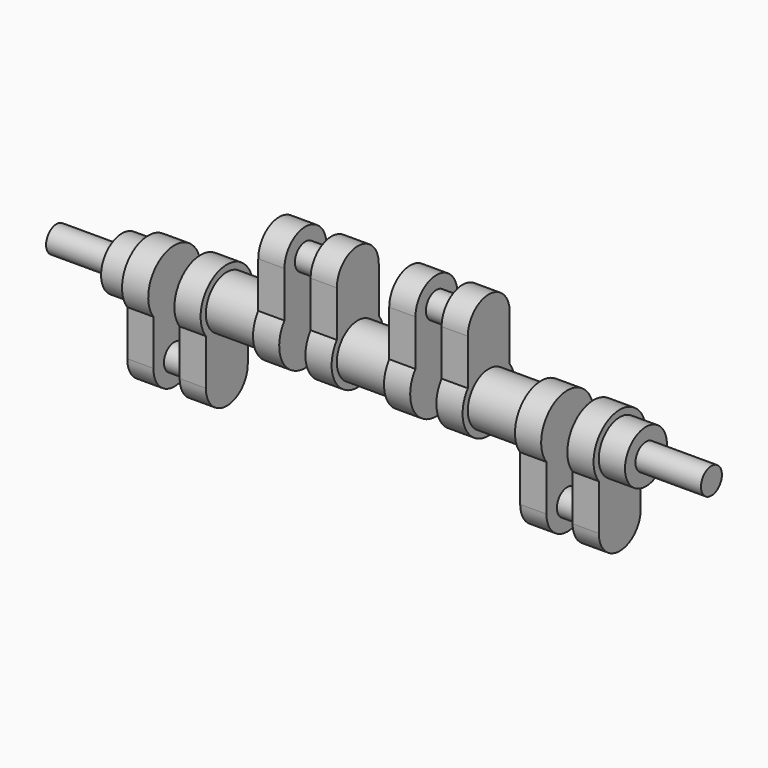
from build123d import *

# Parameters (mm, degrees)
F0_R      = 12.7
F1_DEPTH  = 63.5
F3_R      = 25.4
F4_DEPTH  = 25.4
F6_DEPTH  = 25.4
F7_R      = 12.7
F8_DEPTH  = 25.4
F10_DEPTH = 25.4
F11_R     = 25.4
F12_DEPTH = 50.8
F14_DEPTH = 25.4
F15_R     = 12.7
F16_DEPTH = 25.4
F18_DEPTH = 25.4
F19_R     = 25.4
F20_DEPTH = 50.8
F22_DEPTH = 25.4
F23_R     = 12.7
F24_DEPTH = 25.4
F26_DEPTH = 25.4
F27_R     = 25.4
F28_DEPTH = 50.8
F30_DEPTH = 25.4
F31_R     = 12.7
F32_DEPTH = 25.4
F34_DEPTH = 25.4
F35_R     = 25.4
F36_DEPTH = 25.4
F37_R     = 12.7
F38_DEPTH = 63.5


with BuildPart() as f1:
    # F0 (on Right) → F1 (new body)
    with BuildSketch(Plane.YZ):
        Circle(F0_R)
    extrude(amount=F1_DEPTH)

    # F3 (on face) → F4 (join)
    with BuildSketch(Plane.YZ.offset(63.5)):
        Circle(F3_R)
    extrude(amount=F4_DEPTH)

    # F5 (on face) → F6 (join)
    with BuildSketch(Plane.YZ.offset(88.9)):
        with BuildLine():
            ThreePointArc((25.3964688963, -19.0547072295), (0, -31.75), (-25.3964688963, -19.0547072295))
            Line((-25.3964688963, -19.0547072295), (-25.3964688963, -63.0764818772))
            ThreePointArc((-25.3964688963, -63.0764818772), (0, -38.1), (25.3964688963, -63.0764818772))
            Line((25.3964688963, -63.0764818772), (25.3964688963, -19.0547072295))
        make_face()
        with BuildLine():
            ThreePointArc((31.75, 0), (-10.0430227657, 30.1197641712), (-25.3964688963, -19.0547072295))
            ThreePointArc((-25.3964688963, -19.0547072295), (0, -31.75), (25.3964688963, -19.0547072295))
            ThreePointArc((25.3964688963, -19.0547072295), (30.1197641712, -10.0430227657), (31.75, 0))
        make_face()
        with BuildLine():
            ThreePointArc((25.3964688963, -63.0764818772), (0, -38.1), (-25.3964688963, -63.0764818772))
            Line((-25.3964688963, -63.0764818772), (25.3964688963, -63.9235181228))
            Line((25.3964688963, -63.9235181228), (25.3964688963, -63.0764818772))
        make_face()
        with BuildLine():
            Line((25.3964688963, -63.9235181228), (-25.3964688963, -63.0764818772))
            ThreePointArc((-25.3964688963, -63.0764818772), (-0.4235181228, -88.8964688963), (25.3964688963, -63.9235181228))
        make_face()
        with BuildLine():
            Line((25.3964688963, -63.0764818772), (25.3964688963, -63.9235181228))
            ThreePointArc((25.3964688963, -63.9235181228), (25.3991172087, -63.7117664215), (25.4, -63.5))
            ThreePointArc((25.4, -63.5), (25.3991172087, -63.2882335785), (25.3964688963, -63.0764818772))
        make_face()
    extrude(amount=F6_DEPTH)

    # F7 (on face) → F8 (join)
    with BuildSketch(Plane.YZ.offset(114.3)):
        with Locations((0, -63.5)):
            Circle(F7_R)
    extrude(amount=F8_DEPTH)

    # F9 (on face) → F10 (join)
    with BuildSketch(Plane.YZ.offset(139.7)):
        with BuildLine():
            Line((0, -63.5), (25.4, -63.5))
            ThreePointArc((25.4, -63.5), (0, -38.1), (-25.4, -63.5))
            Line((-25.4, -63.5), (0, -63.5))
        make_face()
        with BuildLine():
            ThreePointArc((-25.4, -63.5), (0, -88.9), (25.4, -63.5))
            Line((25.4, -63.5), (0, -63.5))
            Line((0, -63.5), (-25.4, -63.5))
        make_face()
        with BuildLine():
            ThreePointArc((-25.4, -63.5), (0, -38.1), (25.4, -63.5))
            Line((25.4, -63.5), (25.4, -19.05))
            ThreePointArc((25.4, -19.05), (0, -31.75), (-25.4, -19.05))
            Line((-25.4, -19.05), (-25.4, -63.5))
        make_face()
        with BuildLine():
            ThreePointArc((-25.4, -19.05), (0, -31.75), (25.4, -19.05))
            Line((25.4, -19.05), (25.4, 0))
            ThreePointArc((25.4, 0), (0, -25.4), (-25.4, 0))
            Line((-25.4, 0), (-25.4, -19.05))
        make_face()
        with BuildLine():
            Line((25.4, 0), (25.4, -19.05))
            ThreePointArc((25.4, -19.05), (30.1206947131, -10.040231571), (31.75, 0))
            ThreePointArc((31.75, 0), (-10.040231571, 30.1206947131), (-25.4, -19.05))
            Line((-25.4, -19.05), (-25.4, 0))
            ThreePointArc((-25.4, 0), (0, 25.4), (25.4, 0))
        make_face()
        with BuildLine():
            ThreePointArc((-25.4, 0), (0, -25.4), (25.4, 0))
            ThreePointArc((25.4, 0), (0, 25.4), (-25.4, 0))
        make_face()
    extrude(amount=F10_DEPTH)

    # F11 (on face) → F12 (join)
    with BuildSketch(Plane.YZ.offset(165.1)):
        Circle(F11_R)
    extrude(amount=F12_DEPTH)

    # F13 (on face) → F14 (join)
    with BuildSketch(Plane.YZ.offset(215.9)):
        with BuildLine():
            Line((0, 0), (25.4, 0))
            ThreePointArc((25.4, 0), (0, 25.4), (-25.4, 0))
            Line((-25.4, 0), (0, 0))
        make_face()
        with BuildLine():
            Line((25.4, 19.05), (25.4, 0))
            ThreePointArc((25.4, 0), (0, -25.4), (-25.4, 0))
            Line((-25.4, 0), (-25.4, 19.05))
            ThreePointArc((-25.4, 19.05), (-10.040231571, -30.1206947131), (31.75, 0))
            ThreePointArc((31.75, 0), (30.1206947131, 10.040231571), (25.4, 19.05))
        make_face()
        with BuildLine():
            ThreePointArc((-25.4, 0), (0, -25.4), (25.4, 0))
            Line((25.4, 0), (0, 0))
            Line((0, 0), (-25.4, 0))
        make_face()
        with BuildLine():
            ThreePointArc((-25.4, 0), (0, 25.4), (25.4, 0))
            Line((25.4, 0), (25.4, 19.05))
            ThreePointArc((25.4, 19.05), (0, 31.75), (-25.4, 19.05))
            Line((-25.4, 19.05), (-25.4, 0))
        make_face()
        with BuildLine():
            ThreePointArc((-25.4, 19.05), (0, 31.75), (25.4, 19.05))
            Line((25.4, 19.05), (25.4, 63.5))
            ThreePointArc((25.4, 63.5), (0, 38.1), (-25.4, 63.5))
            Line((-25.4, 63.5), (-25.4, 19.05))
        make_face()
        with BuildLine():
            ThreePointArc((-25.4, 63.5), (0, 38.1), (25.4, 63.5))
            Line((25.4, 63.5), (-25.4, 63.5))
        make_face()
        with BuildLine():
            Line((-25.4, 63.5), (25.4, 63.5))
            ThreePointArc((25.4, 63.5), (0, 88.9), (-25.4, 63.5))
        make_face()
    extrude(amount=F14_DEPTH)

    # F15 (on face) → F16 (join)
    with BuildSketch(Plane.YZ.offset(241.3)):
        with Locations((0, 63.5)):
            Circle(F15_R)
    extrude(amount=F16_DEPTH)

    # F17 (on face) → F18 (join)
    with BuildSketch(Plane.YZ.offset(266.7)):
        with BuildLine():
            Line((-25.4, 63.5), (25.4, 63.5))
            ThreePointArc((25.4, 63.5), (0, 88.9), (-25.4, 63.5))
        make_face()
        with BuildLine():
            Line((25.4, 19.05), (25.4, 63.5))
            ThreePointArc((25.4, 63.5), (0, 38.1), (-25.4, 63.5))
            Line((-25.4, 63.5), (-25.4, 19.05))
            ThreePointArc((-25.4, 19.05), (0, 31.75), (25.4, 19.05))
        make_face()
        with BuildLine():
            ThreePointArc((-25.4, 63.5), (0, 38.1), (25.4, 63.5))
            Line((25.4, 63.5), (-25.4, 63.5))
        make_face()
        with BuildLine():
            ThreePointArc((31.75, 0), (30.1206947131, 10.040231571), (25.4, 19.05))
            Line((25.4, 19.05), (25.4, 0))
            ThreePointArc((25.4, 0), (0, -25.4), (-25.4, 0))
            Line((-25.4, 0), (-25.4, 19.05))
            ThreePointArc((-25.4, 19.05), (-10.040231571, -30.1206947131), (31.75, 0))
        make_face()
        with BuildLine():
            Line((25.4, 0), (25.4, 19.05))
            ThreePointArc((25.4, 19.05), (0, 31.75), (-25.4, 19.05))
            Line((-25.4, 19.05), (-25.4, 0))
            ThreePointArc((-25.4, 0), (0, 25.4), (25.4, 0))
        make_face()
        with BuildLine():
            ThreePointArc((-25.4, 0), (0, -25.4), (25.4, 0))
            ThreePointArc((25.4, 0), (0, 25.4), (-25.4, 0))
        make_face()
    extrude(amount=F18_DEPTH)

    # F19 (on face) → F20 (join)
    with BuildSketch(Plane.YZ.offset(292.1)):
        Circle(F19_R)
    extrude(amount=F20_DEPTH)

    # F21 (on face) → F22 (join)
    with BuildSketch(Plane.YZ.offset(342.9)):
        with BuildLine():
            Line((-25.4, 0), (25.4, 0))
            ThreePointArc((25.4, 0), (0, 25.4), (-25.4, 0))
        make_face()
        with BuildLine():
            ThreePointArc((-25.4, 63.5), (0, 38.1), (25.4, 63.5))
            Line((25.4, 63.5), (-25.4, 63.5))
        make_face()
        with BuildLine():
            Line((25.4, 0), (25.4, 19.05))
            ThreePointArc((25.4, 19.05), (0, 31.75), (-25.4, 19.05))
            Line((-25.4, 19.05), (-25.4, 0))
            ThreePointArc((-25.4, 0), (0, 25.4), (25.4, 0))
        make_face()
        with BuildLine():
            ThreePointArc((-25.4, 19.05), (-10.040231571, -30.1206947131), (31.75, 0))
            ThreePointArc((31.75, 0), (30.1206947131, 10.040231571), (25.4, 19.05))
            Line((25.4, 19.05), (25.4, 0))
            ThreePointArc((25.4, 0), (0, -25.4), (-25.4, 0))
            Line((-25.4, 0), (-25.4, 19.05))
        make_face()
        with BuildLine():
            Line((-25.4, 63.5), (25.4, 63.5))
            ThreePointArc((25.4, 63.5), (0, 88.9), (-25.4, 63.5))
        make_face()
        with BuildLine():
            ThreePointArc((-25.4, 19.05), (0, 31.75), (25.4, 19.05))
            Line((25.4, 19.05), (25.4, 63.5))
            ThreePointArc((25.4, 63.5), (0, 38.1), (-25.4, 63.5))
            Line((-25.4, 63.5), (-25.4, 19.05))
        make_face()
        with BuildLine():
            ThreePointArc((-25.4, 0), (0, -25.4), (25.4, 0))
            Line((25.4, 0), (-25.4, 0))
        make_face()
    extrude(amount=F22_DEPTH)

    # F23 (on face) → F24 (join)
    with BuildSketch(Plane.YZ.offset(368.3)):
        with Locations((0, 63.5)):
            Circle(F23_R)
    extrude(amount=F24_DEPTH)

    # F25 (on face) → F26 (join)
    with BuildSketch(Plane.YZ.offset(393.7)):
        with BuildLine():
            Line((0, 63.5), (25.4, 63.5))
            ThreePointArc((25.4, 63.5), (0, 88.9), (-25.4, 63.5))
            Line((-25.4, 63.5), (0, 63.5))
        make_face()
        with BuildLine():
            Line((25.4, 19.05), (25.4, 63.5))
            ThreePointArc((25.4, 63.5), (0, 38.1), (-25.4, 63.5))
            Line((-25.4, 63.5), (-25.4, 19.05))
            ThreePointArc((-25.4, 19.05), (0, 31.75), (25.4, 19.05))
        make_face()
        with BuildLine():
            ThreePointArc((-25.4, 63.5), (0, 38.1), (25.4, 63.5))
            Line((25.4, 63.5), (0, 63.5))
            Line((0, 63.5), (-25.4, 63.5))
        make_face()
        with BuildLine():
            ThreePointArc((31.75, 0), (30.1206947131, 10.040231571), (25.4, 19.05))
            Line((25.4, 19.05), (25.4, 0))
            Line((25.4, 0), (-25.4, 0))
            Line((-25.4, 0), (-25.4, 19.05))
            ThreePointArc((-25.4, 19.05), (-10.040231571, -30.1206947131), (31.75, 0))
        make_face()
        with BuildLine():
            Line((25.4, 0), (25.4, 19.05))
            ThreePointArc((25.4, 19.05), (0, 31.75), (-25.4, 19.05))
            Line((-25.4, 19.05), (-25.4, 0))
            Line((-25.4, 0), (25.4, 0))
        make_face()
    extrude(amount=F26_DEPTH)

    # F27 (on face) → F28 (join)
    with BuildSketch(Plane.YZ.offset(419.1)):
        Circle(F27_R)
    extrude(amount=F28_DEPTH)

    # F29 (on face) → F30 (join)
    with BuildSketch(Plane.YZ.offset(469.9)):
        with BuildLine():
            ThreePointArc((25.4, -19.05), (30.1206947131, -10.040231571), (31.75, 0))
            ThreePointArc((31.75, 0), (-10.040231571, 30.1206947131), (-25.4, -19.05))
            Line((-25.4, -19.05), (-25.4, 0))
            ThreePointArc((-25.4, 0), (0, 25.4), (25.4, 0))
            Line((25.4, 0), (25.4, -19.05))
        make_face()
        with BuildLine():
            Line((-25.4, 0), (-25.4, -19.05))
            ThreePointArc((-25.4, -19.05), (0, -31.75), (25.4, -19.05))
            Line((25.4, -19.05), (25.4, 0))
            ThreePointArc((25.4, 0), (0, -25.4), (-25.4, 0))
        make_face()
        with BuildLine():
            ThreePointArc((25.4, -19.05), (0, -31.75), (-25.4, -19.05))
            Line((-25.4, -19.05), (-25.4, -63.5))
            ThreePointArc((-25.4, -63.5), (0, -38.1), (25.4, -63.5))
            Line((25.4, -63.5), (25.4, -19.05))
        make_face()
        with BuildLine():
            ThreePointArc((25.4, -63.5), (0, -38.1), (-25.4, -63.5))
            Line((-25.4, -63.5), (25.4, -63.5))
        make_face()
        with BuildLine():
            Line((25.4, -63.5), (-25.4, -63.5))
            ThreePointArc((-25.4, -63.5), (0, -88.9), (25.4, -63.5))
        make_face()
        with BuildLine():
            ThreePointArc((25.4, 0), (0, 25.4), (-25.4, 0))
            Line((-25.4, 0), (25.4, 0))
        make_face()
        with BuildLine():
            Line((25.4, 0), (-25.4, 0))
            ThreePointArc((-25.4, 0), (0, -25.4), (25.4, 0))
        make_face()
    extrude(amount=F30_DEPTH)

    # F31 (on face) → F32 (join)
    with BuildSketch(Plane.YZ.offset(495.3)):
        with Locations((0, -63.5)):
            Circle(F31_R)
    extrude(amount=F32_DEPTH)

    # F33 (on face) → F34 (join)
    with BuildSketch(Plane.YZ.offset(520.7)):
        with BuildLine():
            Line((12.7, -63.5), (25.4, -63.5))
            ThreePointArc((25.4, -63.5), (0, -38.1), (-25.4, -63.5))
            Line((-25.4, -63.5), (-12.7, -63.5))
            ThreePointArc((-12.7, -63.5), (0, -50.8), (12.7, -63.5))
        make_face()
        with BuildLine():
            ThreePointArc((-25.4, -63.5), (0, -88.9), (25.4, -63.5))
            Line((25.4, -63.5), (12.7, -63.5))
            ThreePointArc((12.7, -63.5), (0, -76.2), (-12.7, -63.5))
            Line((-12.7, -63.5), (-25.4, -63.5))
        make_face()
        with BuildLine():
            ThreePointArc((-25.4, -63.5), (0, -38.1), (25.4, -63.5))
            Line((25.4, -63.5), (25.4, -19.05))
            ThreePointArc((25.4, -19.05), (0, -31.75), (-25.4, -19.05))
            Line((-25.4, -19.05), (-25.4, -63.5))
        make_face()
        with BuildLine():
            ThreePointArc((-12.7, -63.5), (0, -76.2), (12.7, -63.5))
            Line((12.7, -63.5), (0, -63.5))
            Line((0, -63.5), (-12.7, -63.5))
        make_face()
        with BuildLine():
            Line((0, -63.5), (12.7, -63.5))
            ThreePointArc((12.7, -63.5), (0, -50.8), (-12.7, -63.5))
            Line((-12.7, -63.5), (0, -63.5))
        make_face()
        with BuildLine():
            ThreePointArc((-25.4, -19.05), (0, -31.75), (25.4, -19.05))
            Line((25.4, -19.05), (25.4, 0))
            ThreePointArc((25.4, 0), (0, -25.4), (-25.4, 0))
            Line((-25.4, 0), (-25.4, -19.05))
        make_face()
        with BuildLine():
            Line((25.4, 0), (25.4, -19.05))
            ThreePointArc((25.4, -19.05), (30.1206947131, -10.040231571), (31.75, 0))
            ThreePointArc((31.75, 0), (-10.040231571, 30.1206947131), (-25.4, -19.05))
            Line((-25.4, -19.05), (-25.4, 0))
            ThreePointArc((-25.4, 0), (0, 25.4), (25.4, 0))
        make_face()
        with BuildLine():
            Line((0, 0), (25.4, 0))
            ThreePointArc((25.4, 0), (0, 25.4), (-25.4, 0))
            Line((-25.4, 0), (0, 0))
        make_face()
        with BuildLine():
            ThreePointArc((-25.4, 0), (0, -25.4), (25.4, 0))
            Line((25.4, 0), (0, 0))
            Line((0, 0), (-25.4, 0))
        make_face()
    extrude(amount=F34_DEPTH)

    # F35 (on face) → F36 (join)
    with BuildSketch(Plane.YZ.offset(546.1)):
        Circle(F35_R)
    extrude(amount=F36_DEPTH)

    # F37 (on face) → F38 (join)
    with BuildSketch(Plane.YZ.offset(571.5)):
        Circle(F37_R)
    extrude(amount=F38_DEPTH)


solid = f1.part
